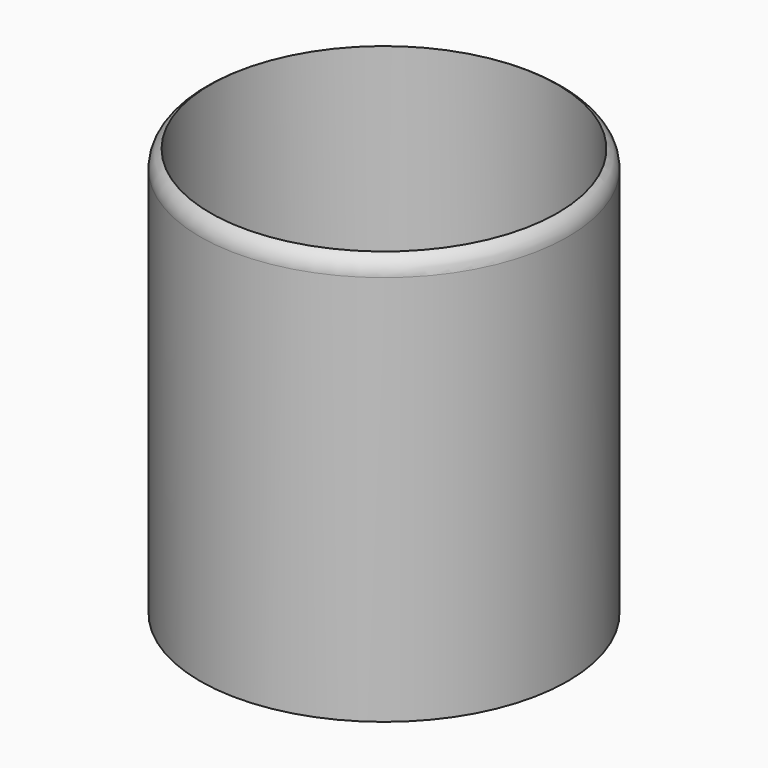
from build123d import *

# Parameters (mm, degrees)
F0_R     = 45
F1_DEPTH = 100
F3_R     = 42.5
F4_DEPTH = 90


# Not quite as in the source:
# - a fillet or chamfer that OpenCascade refuses, or shapes differently, is made with other operations: its cross-section is extruded or revolved along the edge and cut away or added


with BuildPart() as f1:
    # F0 (on Top) → F1 (new body)
    with BuildSketch(Plane.XY):
        Circle(F0_R)
    extrude(amount=F1_DEPTH)

    # F3 (on face) → F4 (cut)
    with BuildSketch(Plane.XY.offset(100)):
        Circle(F3_R)
    extrude(amount=-F4_DEPTH, mode=Mode.SUBTRACT)

    # F5: fillet of radius 5 on 1 edges, made by hand

    # F5_s1 → F5_t2 (revolve, cut)
    with BuildSketch(Plane.XZ):
        with BuildLine():
            ThreePointArc((45, 95.6698729811), (44.3301270189, 98.1698729811), (42.5, 100))
            Line((42.5, 100), (45, 100))
            Line((45, 100), (45, 95.6698729811))
        make_face()
    revolve(axis=Axis((0, 0, 100), (0, 0, 1)), mode=Mode.SUBTRACT)


solid = f1.part
